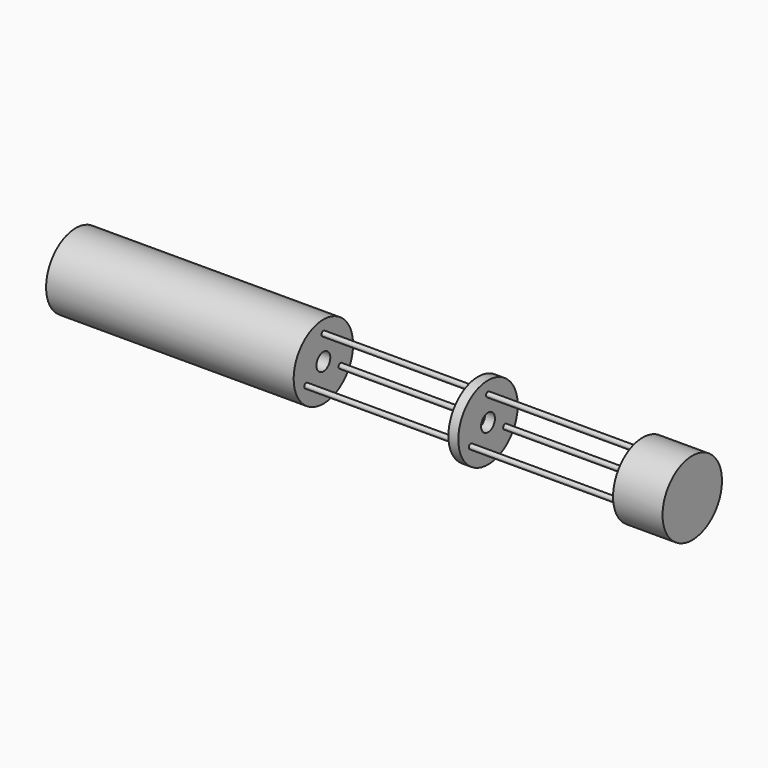
from build123d import *

# Parameters (mm, degrees)
F2_W     = 20
F2_H     = 57.5
F1_W     = 100
F1_H     = 75
F4_R     = 5
F5_DEPTH = 645


# Not quite as in the source:
# - a feature names something its author has since deleted; it is built from what else it names


with BuildPart() as f3:
    # F0 (on Top) → F3 (revolve)
    with BuildSketch(Plane.XY):
        Polygon((-200, 0), (-500, 0), (-500, -75), (0, -75), (0, -17.5), (-200, -17.5), align=None)
    revolve(axis=Axis((-350, 0, 0), (-1, 0, 0)))


with BuildPart() as f3b:
    # F2 (on Top) → F3, piece 2 (revolve)
    with BuildSketch(Plane.XY):
        with Locations((322.5, -46.25)):
            Rectangle(F2_W, F2_H)
    revolve(axis=Axis((-350, 0, 0), (-1, 0, 0)))


with BuildPart() as f3c:
    # F1 (on Top) → F3, piece 3 (revolve)
    with BuildSketch(Plane.XY):
        with Locations((695, -37.5)):
            Rectangle(F1_W, F1_H)
    revolve(axis=Axis((-350, 0, 0), (-1, 0, 0)))


with BuildPart() as f5:
    # F4 (on Right) → F5 (new body, through all)
    with BuildSketch(Plane.YZ):
        with Locations((0, 50)):
            Circle(F4_R)
    extrude(amount=F5_DEPTH)


with BuildPart() as f5b:
    # F4 (on Right) → F5, piece 2 (new body, through all)
    with BuildSketch(Plane.YZ):
        with Locations((-43.3012701892, -25)):
            Circle(F4_R)
    extrude(amount=F5_DEPTH)


with BuildPart() as f5c:
    # F4 (on Right) → F5, piece 3 (new body, through all)
    with BuildSketch(Plane.YZ):
        with Locations((43.3012701892, -25)):
            Circle(F4_R)
    extrude(amount=F5_DEPTH)


solid = Compound([f3.part, f3b.part, f3c.part, f5.part, f5b.part, f5c.part])
